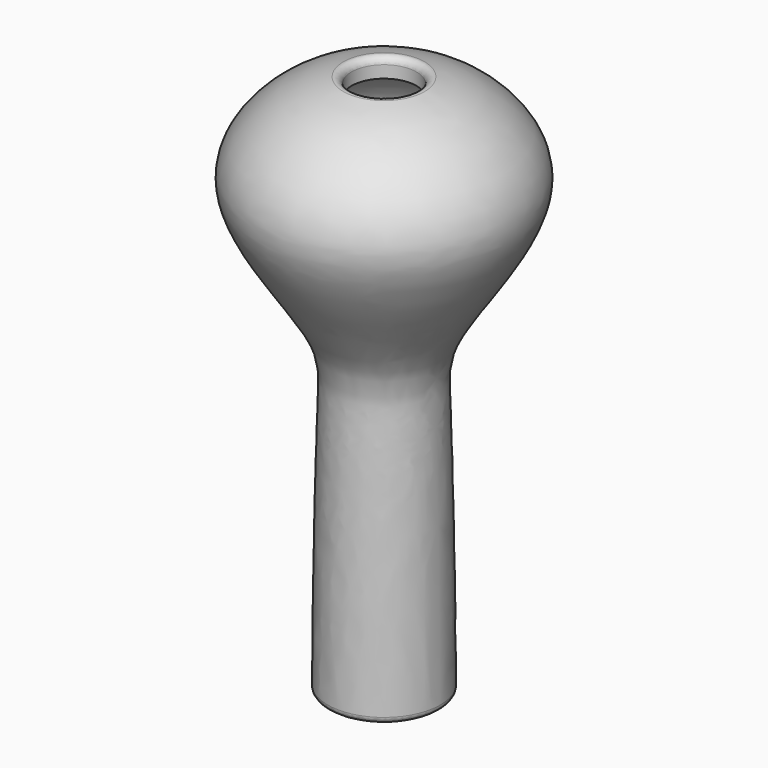
from build123d import *

# Parameters (mm, degrees)
F2_R = 0.3


# Not quite as in the source:
# - the dataset's text gives a spline's control points without its knots; the knots are read off the source's solid


with BuildPart() as f1:
    # F0 (on Front) → F1 (revolve)
    with BuildSketch(Plane.XZ):
        with BuildLine():
            Line((1.6, 12.4103714585), (1.6, 0))
            Line((1.6, 0), (2.6, 0))
            add(Edge.make_bspline(
                [(1.5, 25), (2.9321064445, 24.7354908403), (4.9587102124, 23.7216032659), (7.1308892101, 20.1077407545), (2.2967047813, 14.6507552475), (2.3982847318, 11.4976299192), (2.5386375035, 7.1872878924), (2.6, 0)],
                knots=[0, 0, 0, 0, 0.168662224, 0.3297136611, 0.5545466145, 0.6946432256, 1, 1, 1, 1], degree=3))
            Line((1.5, 25), (1.5, 24.0669772029))
            add(Edge.make_bspline(
                [(1.5, 24.0669772029), (1.9408950233, 23.9687035141), (3.3109616799, 23.7289593916), (5.7653637967, 20.6790738458), (3.5837741417, 17.5236820455), (1.5516486019, 14.8571049795), (1.6, 13.2279656827)],
                knots=[0, 0, 0, 0, 0.1834156363, 0.4351648198, 0.6944218935, 1, 1, 1, 1], degree=3))
            Line((1.6, 13.2279656827), (1.6, 12.4103714585))
        make_face()
        with BuildLine():
            add(Edge.make_bspline(
                [(1.6, 12.4103714585), (1.5823024849, 12.3953360572), (1.4876570216, 12.3162639116), (1.3426761427, 12.2064526867), (1.1553019883, 12.0909653074), (0.9677670698, 11.9909427662), (0.7786558017, 11.9102776458), (0.5920074055, 11.849742975), (0.4020440058, 11.8022001083), (0.1791912103, 11.7772686271), (0.0509296666, 11.7784226274), (0, 11.7784968314)],
                knots=[0.2206760127, 0.2206760127, 0.2206760127, 0.2206760127, 0.25, 0.375, 0.4375, 0.5, 0.625, 0.6875, 0.75, 0.875, 1, 1, 1, 1], degree=3))
            Line((1.6, 12.4103714585), (1.6, 13.2279656827))
            add(Edge.make_bspline(
                [(1.6, 13.2279656827), (1.4113533887, 13.0268188884), (0.9455979841, 12.674075339), (0.3582057912, 12.3702716941), (0.1015206279, 12.3596613094), (0, 12.3546328396)],
                knots=[0, 0, 0, 0, 0.4022216105, 0.750526107, 1, 1, 1, 1], degree=3))
            Line((0, 12.3546328396), (0, 11.7784968314))
        make_face()
    revolve(axis=Axis((0, 0, 12.5), (0, 0, 1)))

    # F2
    f2_edges = [f1.edges().sort_by_distance(p)[0] for p in [
        (-2.6, 0, 0),
        (-1.6, 0, 0),
        (-1.6, 0, 12.410371),
        (0.857025, 0, 11.945386),
        (-1.5, 0, 25),
    ]]
    fillet(f2_edges, radius=F2_R)


solid = f1.part
